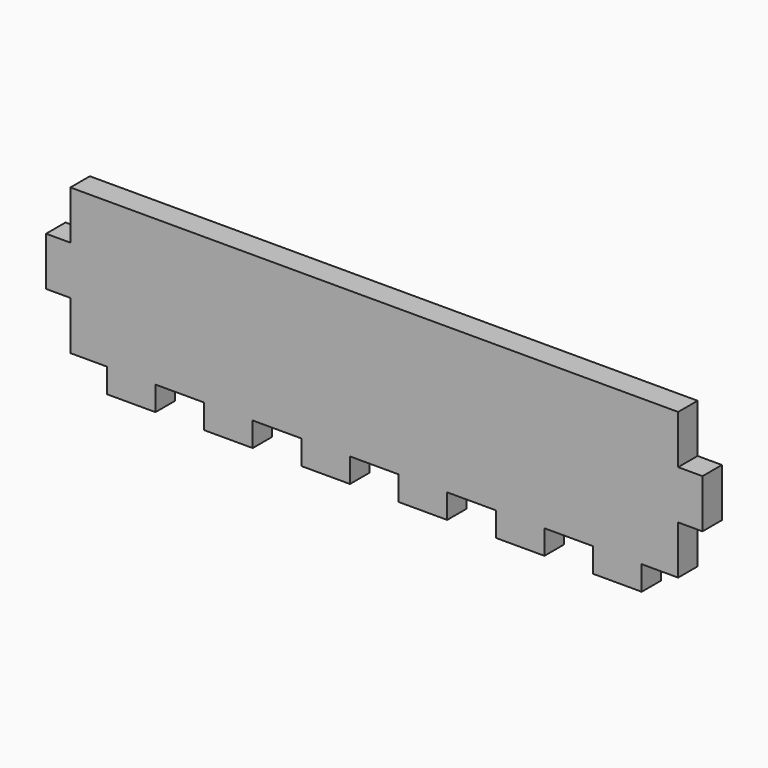
from build123d import *

# Parameters (mm, degrees)
F1_DEPTH = 10


# Not quite as in the source:
# - a feature names something its author has since deleted; it is built from what else it names


with BuildPart() as f1:
    # F0 (on Front) → F1 (new body)
    with BuildSketch(Plane.XZ):
        Polygon((235, 50), (250, 50), (250, 70), (260, 70), (260, 90), (250, 90), (250, 110), (0, 110), (0, 90), (-10, 90), (-10, 70), (0, 70), (0, 50), (15, 50), (15, 40), (35, 40), (35, 50), (55, 50), (55, 40), (75, 40), (75, 50), (95, 50), (95, 40), (115, 40), (115, 50), (135, 50), (135, 40), (155, 40), (155, 50), (175, 50), (175, 40), (195, 40), (195, 50), (215, 50), (215, 40), (235, 40), align=None)
    extrude(amount=-F1_DEPTH)


solid = f1.part
